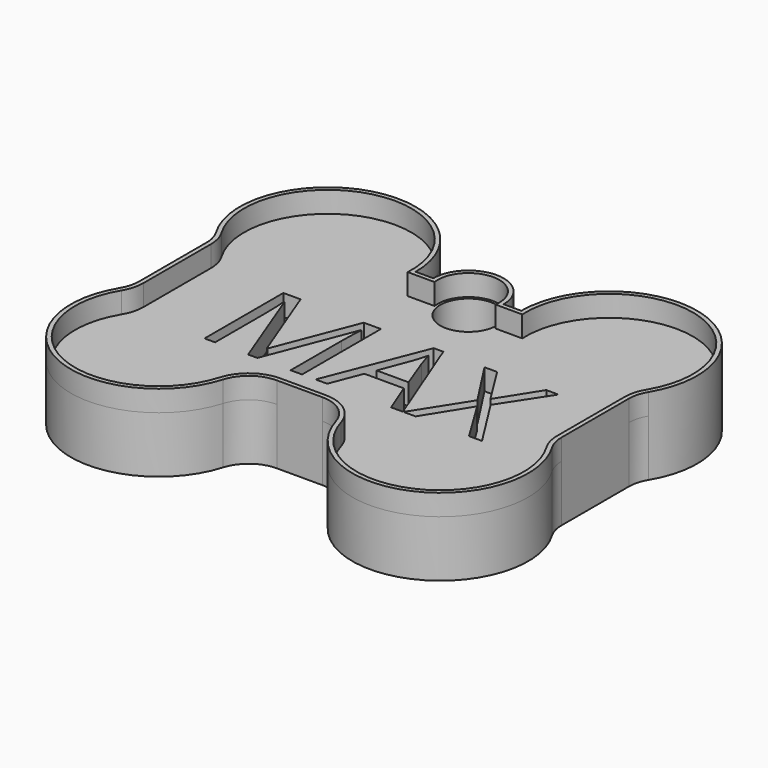
from build123d import *

# Parameters (mm, degrees)
F0_R         = 4
F1_DEPTH     = 8
F2_R         = 5
F3_TEXT_SIZE = 19.6046376063
F4_DEPTH     = 3
F6_DEPTH     = 3


# Not quite as in the source:
# - Text() gives the source's letters only with a copy of the font that has no kerning and outlines rounded to 1/6400 em; it was checked with that copy


with BuildPart() as f1:
    # F0 (on Top) → F1 (new body)
    with BuildSketch(Plane.XY):
        with BuildLine():
            ThreePointArc((0, 7.5), (6.0471529248, -11.8585412256), (22.5, 0))
            Line((22.5, 0), (37.5, 0))
            ThreePointArc((37.5, 0), (53.9528470752, -11.8585412256), (60, 7.5))
            Line((60, 7.5), (60, 22.5))
            ThreePointArc((60, 22.5), (53.9528470752, 41.8585412256), (37.5, 30))
            Line((37.5, 30), (35, 30))
            ThreePointArc((35, 30), (30, 35), (25, 30))
            Line((25, 30), (22.5, 30))
            ThreePointArc((22.5, 30), (6.0471529248, 41.8585412256), (0, 22.5))
            Line((0, 22.5), (0, 7.5))
        make_face()
        with Locations((30, 30)):
            Circle(F0_R, mode=Mode.SUBTRACT)
    extrude(amount=F1_DEPTH)

    # F2
    f2_edges = [f1.edges().sort_by_distance(p)[0] for p in [
        (0, 22.5, 4),
        (0, 7.5, 4),
        (60, 7.5, 4),
        (60, 22.5, 4),
        (22.5, 0, 4),
        (37.5, 0, 4),
    ]]
    fillet(f2_edges, radius=F2_R)

    # F3 (on face) → F4 (cut)
    with BuildSketch(Plane.XY.offset(8)):
        with Locations((8.6922095017, 7.3584682884)):
            Text('MAX', F3_TEXT_SIZE, font='Open Sans', text_align=(TextAlign.LEFT, TextAlign.BOTTOM))
    extrude(amount=-F4_DEPTH, mode=Mode.SUBTRACT)

    # F5 (on face) → F6 (join)
    with BuildSketch(Plane.XY.offset(8)):
        with BuildLine():
            ThreePointArc((0, 9.0138781887), (-0.1818794417, 7.6775719791), (-0.7142857143, 6.4384844205))
            ThreePointArc((-0.7142857143, 6.4384844205), (4.9552577513, -11.4368079307), (21.9789355937, -3.5714285714))
            ThreePointArc((21.9789355937, -3.5714285714), (23.7824383079, -0.9910813713), (26.7705098312, 0))
            Line((26.7705098312, 0), (33.2294901688, 0))
            ThreePointArc((33.2294901688, 0), (36.2175616921, -0.9910813713), (38.0210644063, -3.5714285714))
            ThreePointArc((38.0210644063, -3.5714285714), (55.0447422487, -11.4368079307), (60.7142857143, 6.4384844205))
            ThreePointArc((60.7142857143, 6.4384844205), (60.1818794417, 7.6775719791), (60, 9.0138781887))
            Line((60, 9.0138781887), (60, 20.9861218113))
            ThreePointArc((60, 20.9861218113), (60.1818794417, 22.3224280209), (60.7142857143, 23.5615155795))
            ThreePointArc((60.7142857143, 23.5615155795), (53.3407655239, 42.0453013957), (37.5, 30))
            Line((37.5, 30), (35, 30))
            ThreePointArc((35, 30), (30, 35), (25, 30))
            Line((25, 30), (22.5, 30))
            ThreePointArc((22.5, 30), (6.6592344761, 42.0453013957), (-0.7142857143, 23.5615155795))
            ThreePointArc((-0.7142857143, 23.5615155795), (-0.1818794417, 22.3224280209), (0, 20.9861218113))
            Line((0, 20.9861218113), (0, 9.0138781887))
        make_face()
        with BuildLine():
            ThreePointArc((38.1361902566, 29.3799992651), (52.8751558127, 41.5268322444), (60.1828565129, 23.8808647853))
            ThreePointArc((60.1828565129, 23.8808647853), (59.5844317843, 22.4881301873), (59.3799992651, 20.9861218113))
            Line((59.3799992651, 20.9861218113), (59.3799992651, 9.0138781887))
            ThreePointArc((59.3799992651, 9.0138781887), (59.5844317843, 7.5118698127), (60.1828565129, 6.1191352147))
            ThreePointArc((60.1828565129, 6.1191352147), (54.7945227366, -10.8695415849), (38.615220316, -3.3942855043))
            ThreePointArc((38.615220316, -3.3942855043), (36.5880830002, -0.4939748721), (33.2294901688, 0.6200007349))
            Line((33.2294901688, 0.6200007349), (26.7705098312, 0.6200007349))
            ThreePointArc((26.7705098312, 0.6200007349), (23.4119169998, -0.4939748721), (21.384779684, -3.3942855043))
            ThreePointArc((21.384779684, -3.3942855043), (5.2054772634, -10.8695415849), (-0.1828565129, 6.1191352147))
            ThreePointArc((-0.1828565129, 6.1191352147), (0.4155682157, 7.5118698127), (0.6200007349, 9.0138781887))
            Line((0.6200007349, 9.0138781887), (0.6200007349, 20.9861218113))
            ThreePointArc((0.6200007349, 20.9861218113), (0.4155682157, 22.4881301873), (-0.1828565129, 23.8808647853))
            ThreePointArc((-0.1828565129, 23.8808647853), (7.1248441873, 41.5268322444), (21.8638097434, 29.3799992651))
            Line((21.8638097434, 29.3799992651), (25.6641041698, 29.3799992651))
            ThreePointArc((25.6641041698, 29.3799992651), (30, 34.3799992651), (34.3358958302, 29.3799992651))
            Line((34.3358958302, 29.3799992651), (38.1361902566, 29.3799992651))
        make_face(mode=Mode.SUBTRACT)
    extrude(amount=F6_DEPTH)


solid = f1.part
